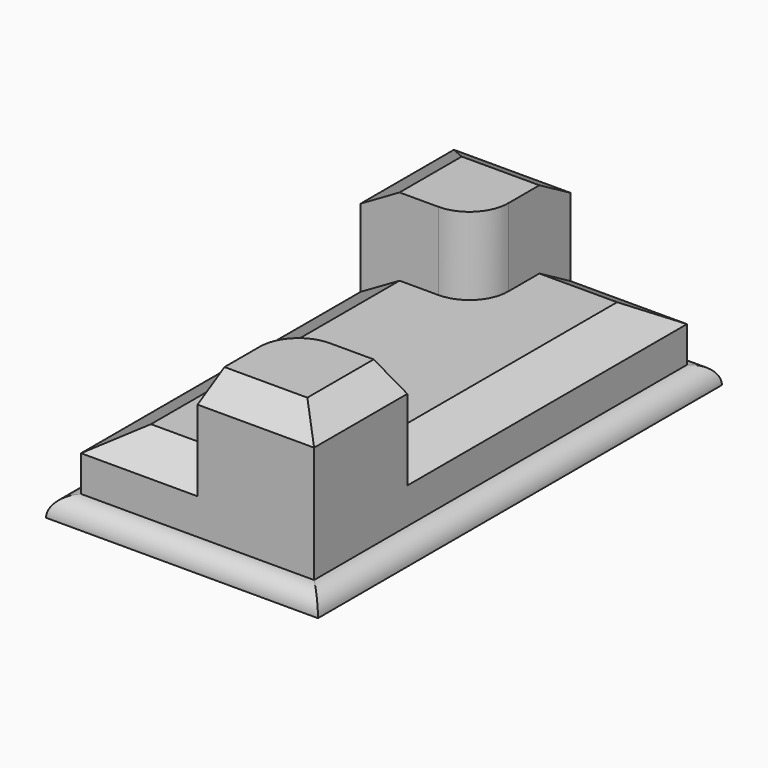
from build123d import *

# Parameters (mm, degrees)
F1_DEPTH = 25.4
F0_W     = 88.9
F0_H     = 165.1
F2_DEPTH = 6.35
F3_DEPTH = 50.8
F4_R     = 6.34999
F5_SIZE2 = 7.3323484187
F5_SIZE  = 12.7
F6_SIZE2 = 7.3323484187
F6_SIZE  = 12.7
F7_SIZE2 = 10.9985226281
F7_SIZE  = 6.35


# Not quite as in the source:
# - a fillet or chamfer is up to 0.001 mm smaller than in the source, because OpenCascade refuses the exact size


with BuildPart() as f1:
    # F0 (on Top) → F1 (new body)
    with BuildSketch(Plane.XY):
        with BuildLine():
            Line((38.1, -38.1), (38.1, 76.2))
            Line((38.1, 76.2), (0, 76.2))
            Line((0, 76.2), (0, 50.8))
            ThreePointArc((0, 50.8), (-3.7197438789, 41.8197438789), (-12.7, 38.1))
            Line((-12.7, 38.1), (-38.1, 38.1))
            Line((-38.1, 38.1), (-38.1, -76.2))
            Line((-38.1, -76.2), (0.0100879326, -76.2))
            Line((0.0100879326, -76.2), (0.0100879326, -50.8))
            ThreePointArc((0.0100879326, -50.8), (3.7298318116, -41.8197438789), (12.7100879326, -38.1))
            Line((12.7100879326, -38.1), (38.1, -38.1))
        make_face()
    extrude(amount=F1_DEPTH)

    # F0 (on Top) → F2 (join)
    with BuildSketch(Plane.XY):
        Rectangle(F0_W, F0_H)
        Polygon((0, 76.2), (38.1, 76.2), (38.1, -38.1), (38.1, -76.2), (0.0100879326, -76.2), (-38.1, -76.2), (-38.1, 38.1), (-38.1, 76.2), align=None, mode=Mode.SUBTRACT)
    extrude(amount=F2_DEPTH)

    # F0 (on Top) → F3 (join)
    with BuildSketch(Plane.XY):
        with BuildLine():
            Line((0, 50.8), (0, 76.2))
            Line((0, 76.2), (-38.1, 76.2))
            Line((-38.1, 76.2), (-38.1, 38.1))
            Line((-38.1, 38.1), (-12.7, 38.1))
            ThreePointArc((-12.7, 38.1), (-3.7197438789, 41.8197438789), (0, 50.8))
        make_face()
        with BuildLine():
            Line((38.1, -76.2), (38.1, -38.1))
            Line((38.1, -38.1), (12.7100879326, -38.1))
            ThreePointArc((12.7100879326, -38.1), (3.7298318116, -41.8197438789), (0.0100879326, -50.8))
            Line((0.0100879326, -50.8), (0.0100879326, -76.2))
            Line((0.0100879326, -76.2), (38.1, -76.2))
        make_face()
    extrude(amount=F3_DEPTH)

    # F4 (radius 6.35 in the source; OpenCascade refuses exactly that, so slightly less here)
    f4_edges = [f1.edges().sort_by_distance(p)[0] for p in [
        (44.45, 0, 6.35),
        (0, 82.55, 6.35),
        (-44.45, 0, 6.35),
        (0, -82.55, 6.35),
    ]]
    fillet(f4_edges, radius=F4_R)

    # F5
    f5_edges = [f1.edges().sort_by_distance(p)[0] for p in [
        (-38.1, -19.05, 25.4),
        (-19.044956, -76.2, 25.4),
        (19.05, 76.2, 25.4),
        (38.1, 19.05, 25.4),
    ]]
    f5_side = f1.faces().sort_by_distance((4e-05, -0.002502, 25.4))[0]
    chamfer(f5_edges, length=F5_SIZE, length2=F5_SIZE2, reference=f5_side)

    # F6
    f6_edges = [f1.edges().sort_by_distance(p)[0] for p in [
        (-38.1, 57.15, 50.8),
        (-19.05, 76.2, 50.8),
    ]]
    f6_side = f1.faces().sort_by_distance((-19.446042, 57.546042, 50.8))[0]
    chamfer(f6_edges, length=F6_SIZE, length2=F6_SIZE2, reference=f6_side)

    # F7
    f7_edges = [f1.edges().sort_by_distance(p)[0] for p in [
        (38.1, -57.15, 50.8),
        (19.055044, -76.2, 50.8),
    ]]
    chamfer(f7_edges, length=F7_SIZE, length2=F7_SIZE2)


solid = f1.part
